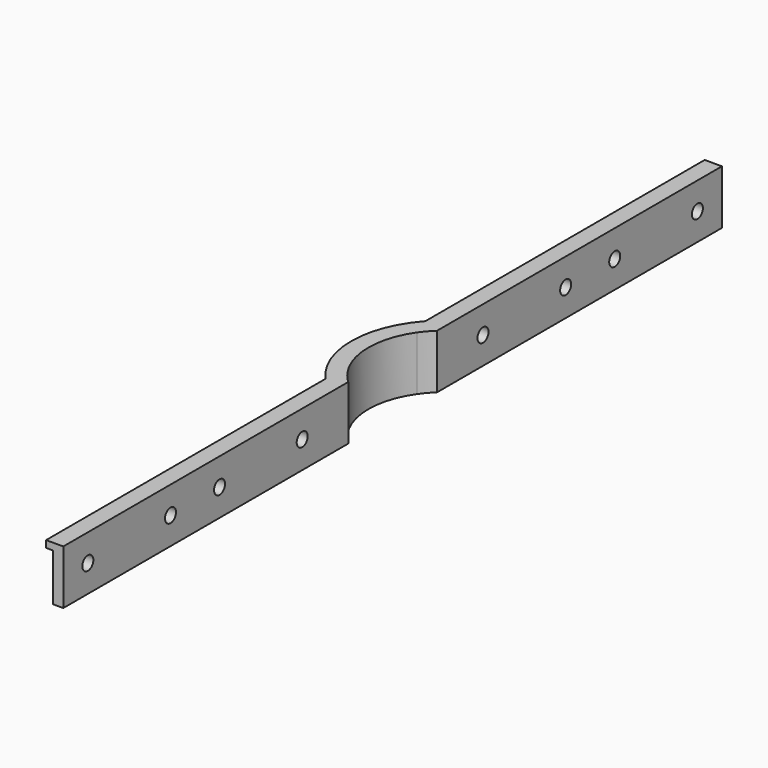
from build123d import *

# Parameters (mm, degrees)
F1_DEPTH = 15.75
F2_R     = 2
F4_DEPTH = 3.001
F3_R     = 2
F5_DEPTH = 3.001
F7_DEPTH = 2


# Not quite as in the source:
# - a feature names something its author has since deleted; it is built from what else it names


with BuildPart() as f1:
    # F0 (on Top) → F1 (new body)
    with BuildSketch(Plane.XY):
        with BuildLine():
            Line((-15, 119.5), (-18, 119.5))
            Line((-18, 119.5), (-18, 17.3493515729))
            ThreePointArc((-18, 17.3493515729), (-25, 0), (-18, -17.3493515729))
            Line((-18, -17.3493515729), (-18, -119.5))
            Line((-18, -119.5), (-15, -119.5))
            Line((-15, -119.5), (-15, -16.0934769394))
            ThreePointArc((-15, -16.0934769394), (-16.5896327506, -14.4493627956), (-18, -12.6491106407))
            ThreePointArc((-18, -12.6491106407), (-22, 0), (-18, 12.6491106407))
            ThreePointArc((-18, 12.6491106407), (-16.5896327506, 14.4493627956), (-15, 16.0934769394))
            Line((-15, 16.0934769394), (-15, 119.5))
        make_face()
    extrude(amount=F1_DEPTH)

    # F2 (on face) → F4 (cut, through all)
    with BuildSketch(Plane(origin=(-18, 0, 0), x_dir=(0, -1, 0), z_dir=(-1, 0, 0))):
        with Locations((-110.6, 7.875)):
            Circle(F2_R)
        with Locations((-80.6, 7.875)):
            Circle(F2_R)
        with Locations((-62.8, 7.875)):
            Circle(F2_R)
        with Locations((-32.8, 7.875)):
            Circle(F2_R)
    extrude(amount=-F4_DEPTH, mode=Mode.SUBTRACT)

    # F3 (on face) → F5 (cut, through all)
    with BuildSketch(Plane(origin=(-18, 0, 0), x_dir=(0, -1, 0), z_dir=(-1, 0, 0))):
        with Locations((32.8, 7.875)):
            Circle(F3_R)
        with Locations((62.8, 7.875)):
            Circle(F3_R)
        with Locations((80.6, 7.875)):
            Circle(F3_R)
        with Locations((110.6, 7.875)):
            Circle(F3_R)
    extrude(amount=-F5_DEPTH, mode=Mode.SUBTRACT)

    # F6 (on face) → F7 (join)
    with BuildSketch(Plane.XY.offset(15.75)):
        with BuildLine():
            ThreePointArc((-20, 18.1383571472), (-27, 0), (-20, -18.1383571472))
            Line((-20, -18.1383571472), (-20, -119.5))
            Line((-20, -119.5), (-18, -119.5))
            Line((-18, -119.5), (-18, -17.3493515729))
            ThreePointArc((-18, -17.3493515729), (-25, 0), (-18, 17.3493515729))
            Line((-18, 17.3493515729), (-18, 119.5))
            Line((-18, 119.5), (-20, 119.5))
            Line((-20, 119.5), (-20, 18.1383571472))
        make_face()
    extrude(amount=-F7_DEPTH)


solid = f1.part
